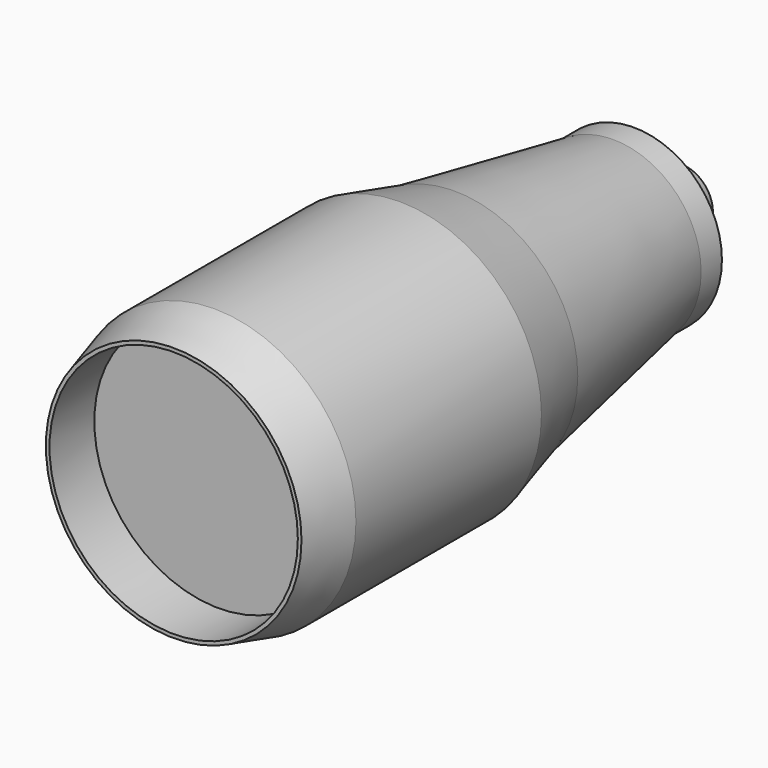
from build123d import *

# Parameters (mm, degrees)
F0_R          = 26.3014880092
F0_R_2        = 23.0827140561
F1_DEPTH      = 39.878
F1_DEPTH_BACK = 25.4
F2_DEPTH      = 14.986
F3_DEPTH      = 76.708
F5_SIZE2      = 3.4029547439
F5_SIZE       = 12.7
F6_SIZE2      = 9.4794090512
F6_SIZE       = 2.54
F7_R          = 13.5748533888
F8_DEPTH      = 15.748
F10_T         = -2.54
F11_DEPTH     = 4.826


# Not quite as in the source:
# - a fillet or chamfer that OpenCascade refuses, or shapes differently, is made with other operations: its cross-section is extruded or revolved along the edge and cut away or added


with BuildPart() as f1:
    # F0 (on Front) → F1 (new body, two sides)
    with BuildSketch(Plane.XZ) as f1_sk:
        Circle(F0_R)
        Circle(F0_R_2, mode=Mode.SUBTRACT)
    extrude(amount=-F1_DEPTH)
    extrude(f1_sk.sketch, amount=F1_DEPTH_BACK)

    # F0 (on Front) → F2 (join)
    with BuildSketch(Plane.XZ):
        Circle(F0_R_2)
    extrude(amount=F2_DEPTH)

    # F0 (on Front) → F3 (join)
    with BuildSketch(Plane.XZ):
        Circle(F0_R_2)
    extrude(amount=-F3_DEPTH)

    # F4: chamfer of 38.1 x 6.718057965 on 1 edges, made by hand


with BuildPart() as f4_tool2:
    # F4_s3 → F4_t4 (revolve)
    with BuildSketch(Plane.XY):
        Polygon((23.0827140561, 38.608), (16.3646560911, 76.708), (23.0827140561, 76.708), align=None)
    revolve(axis=Axis((0, 76.708, 0), (0, -1, 0)))

    split(bisect_by=Plane.XZ.offset(-39.878), keep=Keep.BOTTOM)


with BuildPart() as f1_1:
    add(f1.part)

    # F4_t1: cut F4_tool2
    add(f4_tool2.part, mode=Mode.SUBTRACT)

    # F5
    f5_edges = [f1_1.edges().sort_by_distance(p)[0] for p in [
        (-26.301488, 39.878, 0),
    ]]
    f5_side = f1_1.faces().sort_by_distance((-26.301488, 7.239, 0))[0]
    chamfer(f5_edges, length=F5_SIZE, length2=F5_SIZE2, reference=f5_side)

    # F6
    f6_edges = [f1_1.edges().sort_by_distance(p)[0] for p in [
        (-26.301488, -25.4, 0),
    ]]
    f6_side = f1_1.faces().sort_by_distance((-25.55757, -25.4, 0))[0]
    chamfer(f6_edges, length=F6_SIZE, length2=F6_SIZE2, reference=f6_side)

    # F7 (on face) → F8 (join)
    with BuildSketch(Plane(origin=(0, 76.708, 0), x_dir=(-1, 0, 0), z_dir=(0, 1, 0))):
        Circle(F7_R)
    extrude(amount=F8_DEPTH)

    # F9: chamfer of 7.62 x 28.4382271537 on 1 edges, made by hand


with BuildPart() as f9_tool2:
    # F9_s3 → F9_t4 (revolve)
    with BuildSketch(Plane.XY):
        Polygon((-13.5748533888, 64.0177728463), (-5.9548533888, 92.456), (-13.5748533888, 92.456), align=None)
    revolve(axis=Axis((0, 92.456, 0), (0, 1, 0)))

    split(bisect_by=Plane.XZ.offset(-76.708), keep=Keep.BOTTOM)


with BuildPart() as f1_2:
    add(f1_1.part)

    # F9_t1: cut F9_tool2
    add(f9_tool2.part, mode=Mode.SUBTRACT)

    # F10
    f10_openings = [f1_2.faces().sort_by_distance(p)[0] for p in [
        (0, 92.456, 0),
    ]]
    offset(amount=F10_T, openings=f10_openings, kind=Kind.INTERSECTION)

    # F11 (add): a face of the model
    f11_faces = [f1_2.faces().sort_by_distance(p)[0] for p in [
        (-15.9017937193, 76.708, 0),
    ]]
    extrude(f11_faces, amount=F11_DEPTH)


solid = f1_2.part
